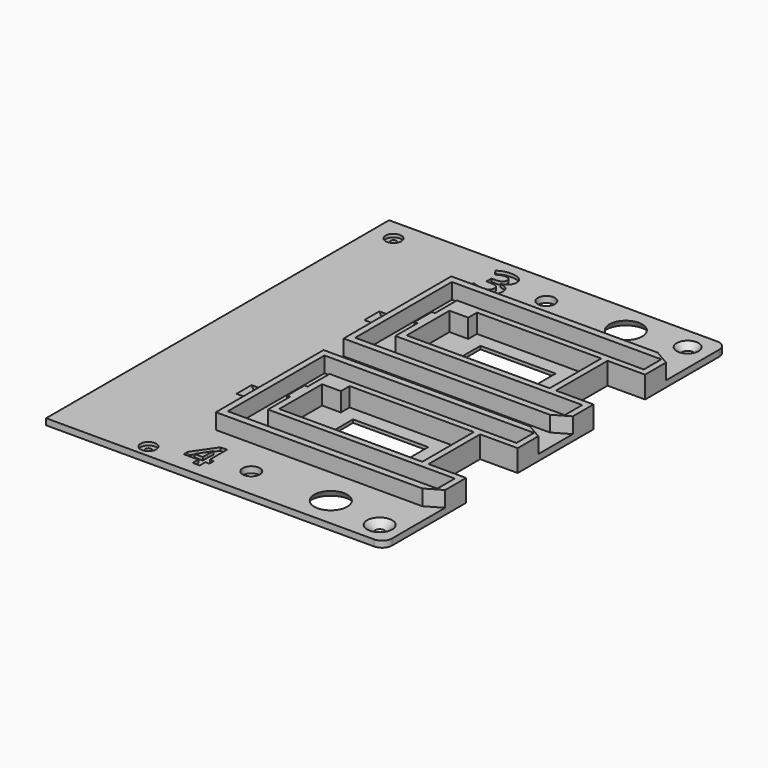
from build123d import *

# Parameters (mm, degrees)
F1_W            = 108
F1_H            = 137
F2_DEPTH        = 2
F3_W            = 70.94
F3_H            = 43
F4_DEPTH        = 5
F5_R            = 5.25
F5_R_2          = 2.75
F5_W            = 10
F5_H            = 20.6
F5_W_2          = 24
F5_H_2          = 11
F6_DEPTH        = 2
F7_R            = 1
F8_DEPTH        = 2
F9_R            = 3.175
F10_TEXT_SIZE   = 17.3078600715
F10_TEXT_SIZE_2 = 15.2777777778
F11_DEPTH       = 1
F12_W           = 8
F12_H           = 9
F12_W_2         = 6.5174393822
F12_H_2         = 20.6
F12_W_3         = 15.5694368295
F13_DEPTH       = 7.001
F15_R           = 3.5
F14_R           = 1.8119398784
F18_R           = 1.5
F17_R           = 4
F20_R           = 2.5
F21_DEPTH       = 1
F23_DEPTH       = 1
F25_DEPTH       = 0.5
F26_W           = 4
F26_H           = 5
F27_DEPTH       = 2.0010001
F28_W           = 5.7
F28_H           = 6
F29_DEPTH       = 2.0010001
F31_DEPTH       = 6
F33_DEPTH       = 6
F34_R           = 5.25
F35_R           = 6.5
F37_R           = 5.25
F38_R           = 6.5
F40_W           = 1
F40_H           = 1
F41_DEPTH       = 5
F42_W           = 8.8
F42_H           = 1.4
F43_DEPTH       = 6
F44_W           = 5
F44_H           = 1
F45_DEPTH       = 1
F47_DEPTH       = 5


# Not quite as in the source:
# - a feature names something its author has since deleted; it is built from what else it names
# - Text() gives the source's letters only with a copy of the font that has no kerning and outlines rounded to 1/6400 em; it was checked with that copy


with BuildPart() as f2:
    # F1 (on Top) → F2 (new body)
    with BuildSketch(Plane.XY):
        with Locations((-54, 68.5)):
            Rectangle(F1_W, F1_H)
    extrude(amount=F2_DEPTH)

    # F3 (on face) → F4 (join)
    with BuildSketch(Plane.XY.offset(2)):
        with Locations((-35.47, 94)):
            Rectangle(F3_W, F3_H)
        Polygon((-68.94, 74.64), (-68.94, 113.24), (-2, 113.24), (-2, 106.24), (-2, 104.24), (-2, 83.64), (-2, 81.64), (-2, 74.64), align=None, mode=Mode.SUBTRACT)
        Polygon((0, 23.76), (0, 62.36), (0, 64.5), (-70.94, 64.5), (-70.94, 21.5), (0, 21.5), align=None)
        Polygon((-68.94, 23.76), (-68.94, 62.36), (-2, 62.36), (-2, 55.36), (-2, 53.36), (-2, 32.76), (-2, 30.76), (-2, 23.76), align=None, mode=Mode.SUBTRACT)
        Polygon((-2, 104.24), (-2, 106.24), (-61.7, 106.24), (-61.7, 81.64), (-2, 81.64), (-2, 83.64), (-12, 83.64), (-12, 104.24), align=None)
        Polygon((-22.8, 102.84), (-14, 102.84), (-14, 83.64), (-51.7, 83.64), (-51.7, 92.64), (-59.7, 92.64), (-59.7, 100.74), (-53.7, 100.74), (-53.7, 104.24), (-22.8, 104.24), align=None, mode=Mode.SUBTRACT)
        Polygon((-2, 53.36), (-2, 55.36), (-61.7, 55.36), (-61.7, 30.76), (-2, 30.76), (-2, 32.76), (-12, 32.76), (-12, 53.36), align=None)
        Polygon((-22.8, 51.96), (-14, 51.96), (-14, 32.76), (-51.7, 32.76), (-51.7, 41.76), (-59.7, 41.76), (-59.7, 49.86), (-53.7, 49.86), (-53.7, 53.36), (-22.8, 53.36), align=None, mode=Mode.SUBTRACT)
    extrude(amount=F4_DEPTH)

    # F5 (on face) → F6 (cut)
    with BuildSketch(Plane.XY.offset(2)):
        with Locations((-24.7, 127.42)):
            Circle(F5_R)
        with Locations((-50.1, 127.42)):
            Circle(F5_R_2)
        with Locations((-24.7, 9.58)):
            Circle(F5_R)
        with Locations((-50.1, 9.58)):
            Circle(F5_R_2)
        with Locations((-7, 93.94)):
            Rectangle(F5_W, F5_H)
        with Locations((-7, 43.06)):
            Rectangle(F5_W, F5_H)
        with Locations((-37, 94.24)):
            Rectangle(F5_W_2, F5_H_2)
        with Locations((-37, 43.36)):
            Rectangle(F5_W_2, F5_H_2)
    extrude(amount=-F6_DEPTH, mode=Mode.SUBTRACT)

    # F7 (on face) → F8 (cut)
    with BuildSketch(Plane.XY.offset(2)):
        with Locations((-101, 130)):
            Circle(F7_R)
        with Locations((-78.5, 4)):
            Circle(F7_R)
    extrude(amount=-F8_DEPTH, mode=Mode.SUBTRACT)

    # F9
    f9_edges = [f2.edges().sort_by_distance(p)[0] for p in [
        (0, 137, 1),
        (0, 0, 1),
    ]]
    fillet(f9_edges, radius=F9_R)

    # F10 (on face) → F11 (cut)
    with BuildSketch(Plane.XY.offset(2)):
        with Locations((-70.94, 121)):
            Text('3', F10_TEXT_SIZE, font='Open Sans', font_style=FontStyle.BOLD, text_align=(TextAlign.LEFT, TextAlign.BOTTOM))
        with Locations((-69.2909114583, 4)):
            Text('4', F10_TEXT_SIZE_2, font='Open Sans', font_style=FontStyle.BOLD, text_align=(TextAlign.LEFT, TextAlign.BOTTOM))
    extrude(amount=-F11_DEPTH, mode=Mode.SUBTRACT)

    # F12 (on face) → F13 (cut, through all)
    with BuildSketch(Plane.XY.offset(7)):
        with Locations((-55.7, 88.14)):
            Rectangle(F12_W, F12_H)
        with Locations((-55.7, 37.26)):
            Rectangle(F12_W, F12_H)
        with Locations((-1.1924867285, 93.94)):
            Rectangle(F12_W_2, F12_H_2)
        with Locations((1.5231149737, 43.06)):
            Rectangle(F12_W_3, F12_H_2)
    extrude(amount=-F13_DEPTH, mode=Mode.SUBTRACT)

    # F15 (on face) → F16 section 0
    with BuildSketch(Plane.XY.offset(2)):
        with Locations((-7, 130)):
            Circle(F15_R)
    # F14 (on face) → F16 section 1
    with BuildSketch(Plane(origin=(0, 0, 0), x_dir=(1, 0, 0), z_dir=(0, 0, -1))):
        with Locations((-7, -130)):
            Circle(F14_R)
    loft(mode=Mode.SUBTRACT)

    # F18 (on face) → F19 section 0
    with BuildSketch(Plane(origin=(0, 0, 0), x_dir=(1, 0, 0), z_dir=(0, 0, -1))):
        with Locations((-7, -7)):
            Circle(F18_R)
    # F17 (on face) → F19 section 1
    with BuildSketch(Plane.XY.offset(2)):
        with Locations((-7, 7)):
            Circle(F17_R)
    loft(mode=Mode.SUBTRACT)

    # F20 (on face) → F21 (cut)
    with BuildSketch(Plane.XY.offset(2)):
        with Locations((-101, 130)):
            Circle(F20_R)
        with Locations((-78.5, 4)):
            Circle(F20_R)
    extrude(amount=-F21_DEPTH, mode=Mode.SUBTRACT)

    # F22 (on face) → F23 (cut)
    with BuildSketch(Plane.XY.offset(2)):
        Polygon((-53.7, 104.24), (-53.7, 100.74), (-59.7, 100.74), (-59.7, 83.64), (-14, 83.64), (-14, 102.84), (-22.8, 102.84), (-22.8, 104.24), align=None)
        Polygon((-22.8, 53.36), (-53.7, 53.36), (-53.7, 49.86), (-59.7, 49.86), (-59.7, 32.76), (-14, 32.76), (-14, 51.96), (-22.8, 51.96), align=None)
    extrude(amount=-F23_DEPTH, mode=Mode.SUBTRACT)

    # F24 (on face) → F25 (cut)
    with BuildSketch(Plane(origin=(0, 0, 0), x_dir=(1, 0, 0), z_dir=(0, 0, -1))):
        Polygon((-82, -50), (-103, -50), (-103, -86.5), (-82, -86.5), (-82, -68.5), align=None)
        Polygon((-102.5, -86), (-102.5, -50.5), (-82.5, -50.5), (-82.5, -75.5), (-82.5, -86), align=None, mode=Mode.SUBTRACT)
    extrude(amount=-F25_DEPTH, mode=Mode.SUBTRACT)

    # F26 (on face) → F27 (cut, through all)
    with BuildSketch(Plane.XY.offset(2)):
        with Locations((-63.7, 43.06)):
            Rectangle(F26_W, F26_H)
        with Locations((-63.7, 93.94)):
            Rectangle(F26_W, F26_H)
    extrude(amount=-F27_DEPTH, mode=Mode.SUBTRACT)

    # F28 (on face) → F29 (cut, through all)
    with BuildSketch(Plane.XY.offset(2)):
        with Locations((-76.29, 94)):
            Rectangle(F28_W, F28_H)
        with Locations((-76.29, 43)):
            Rectangle(F28_W, F28_H)
    extrude(amount=-F29_DEPTH, mode=Mode.SUBTRACT)

    # F30 (on face) → F31 (join)
    with BuildSketch(Plane(origin=(0, 91, 0), x_dir=(-1, 0, 0), z_dir=(0, 1, 0))):
        Polygon((79.14, 0), (79.14, 2), (77.9852994616, 0), align=None)
    extrude(amount=F31_DEPTH)

    # F32 (on face) → F33 (join)
    with BuildSketch(Plane(origin=(0, 40, 0), x_dir=(-1, 0, 0), z_dir=(0, 1, 0))):
        Polygon((77.9852994616, 0), (79.14, 0), (79.14, 2), align=None)
    extrude(amount=F33_DEPTH)

    # F34 (on face) → F36 section 0
    with BuildSketch(Plane.XY.offset(2)):
        with Locations((-24.7, 127.42)):
            Circle(F34_R)
    # F35 (on face) → F36 section 1
    with BuildSketch(Plane(origin=(0, 0, 0), x_dir=(1, 0, 0), z_dir=(0, 0, -1))):
        with Locations((-24.7, -127.42)):
            Circle(F35_R)
    loft(mode=Mode.SUBTRACT)

    # F37 (on face) → F39 section 0
    with BuildSketch(Plane.XY.offset(2)):
        with Locations((-24.7, 9.58)):
            Circle(F37_R)
    # F38 (on face) → F39 section 1
    with BuildSketch(Plane(origin=(0, 0, 0), x_dir=(1, 0, 0), z_dir=(0, 0, -1))):
        with Locations((-24.7, -9.58)):
            Circle(F38_R)
    loft(mode=Mode.SUBTRACT)

    # F40 (on face) → F41 (join)
    with BuildSketch(Plane.XY.offset(2)):
        with Locations((-62.2, 96.94)):
            Rectangle(F40_W, F40_H)
        with Locations((-62.2, 90.94)):
            Rectangle(F40_W, F40_H)
        with Locations((-62.2, 46.06)):
            Rectangle(F40_W, F40_H)
        with Locations((-62.2, 40.06)):
            Rectangle(F40_W, F40_H)
    extrude(amount=F41_DEPTH)

    # F42 (on face) → F43 (cut)
    with BuildSketch(Plane.XY.offset(7)):
        with Locations((-18.4, 103.54)):
            Rectangle(F42_W, F42_H)
        with Locations((-18.4, 52.66)):
            Rectangle(F42_W, F42_H)
    extrude(amount=-F43_DEPTH, mode=Mode.SUBTRACT)

    # F44 (on face) → F45 (join)
    with BuildSketch(Plane(origin=(-61.7, 0, 0), x_dir=(0, -1, 0), z_dir=(-1, 0, 0))):
        with Locations((-93.94, 6.5)):
            Rectangle(F44_W, F44_H)
        with Locations((-43.06, 6.5)):
            Rectangle(F44_W, F44_H)
    extrude(amount=F45_DEPTH)

    # F46 (on face) → F47 (cut)
    with BuildSketch(Plane.XY.offset(7)):
        Polygon((0, 115.5), (-5, 115.5), (0, 112.6132486541), align=None)
        Polygon((0, 72.5), (0, 75.3867513459), (-5, 72.5), align=None)
        Polygon((0, 64.5), (-5, 64.5), (0, 61.6132486541), align=None)
        Polygon((0, 21.5), (0, 24.3867513459), (-5, 21.5), align=None)
    extrude(amount=-F47_DEPTH, mode=Mode.SUBTRACT)


solid = f2.part
